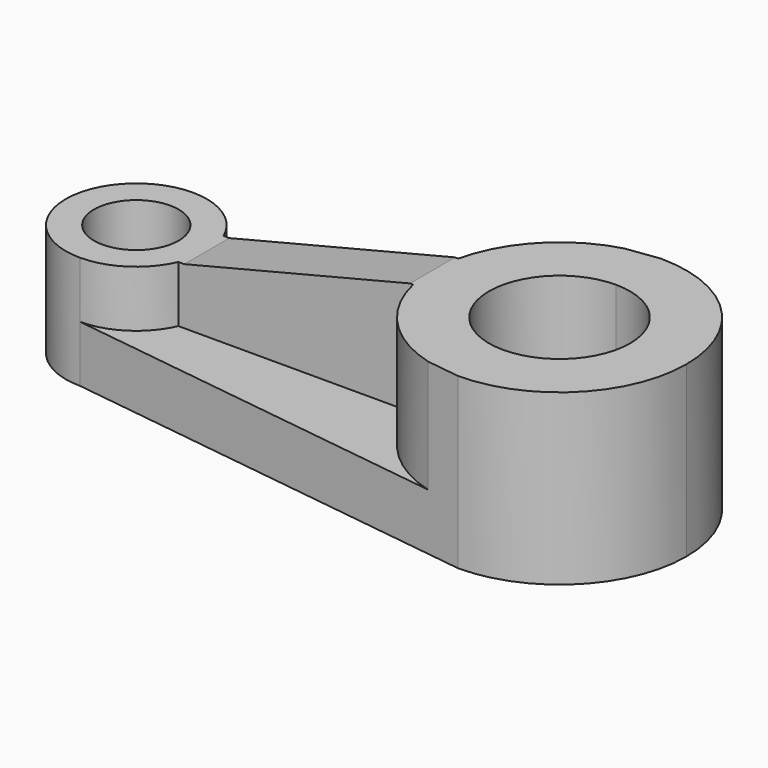
from build123d import *

# Parameters (mm, degrees)
F1_DEPTH = 25.4
F2_DEPTH = 38.1
F3_DEPTH = 12.7
F5_DEPTH = 6.35


with BuildPart() as f1:
    # F0 (on Top) → F1 (new body)
    with BuildSketch(Plane.XY):
        with BuildLine():
            ThreePointArc((-50.8001835883, 0), (-55.449863437, 11.2253201513), (-66.6751835883, 15.875))
            Line((-66.6751835883, 15.875), (-66.6751835883, 9.525))
            ThreePointArc((-66.6751835883, 9.525), (-59.9399914975, 6.7351920908), (-57.1501835883, 0))
            ThreePointArc((-57.1501835883, 0), (-59.9399914975, -6.7351920908), (-66.6751835883, -9.525))
            Line((-66.6751835883, -9.525), (-66.6751835883, -15.875))
            ThreePointArc((-66.6751835883, -15.875), (-55.449863437, -11.2253201513), (-50.8001835883, 0))
        make_face()
        with BuildLine():
            Line((-66.6751835883, 9.525), (-66.6751835883, 15.875))
            ThreePointArc((-66.6751835883, 15.875), (-82.5501835883, 0), (-66.6751835883, -15.875))
            Line((-66.6751835883, -15.875), (-66.6751835883, -9.525))
            ThreePointArc((-66.6751835883, -9.525), (-76.2001835883, 0), (-66.6751835883, 9.525))
        make_face()
    extrude(amount=F1_DEPTH)



with BuildPart() as f2:
    # F0 (on Top) → F2 (new body)
    with BuildSketch(Plane.XY):
        with BuildLine():
            ThreePointArc((28.5748164117, -15.875), (12.6998164117, 0), (28.5748164117, 15.875))
            Line((28.5748164117, 15.875), (28.5748164117, 28.575))
            Line((28.5748164117, 28.575), (21.0879168484, 27.5767467249))
            ThreePointArc((21.0879168484, 27.5767467249), (-0.0001835883, 0), (21.0879168484, -27.5767467249))
            Line((21.0879168484, -27.5767467249), (28.5748164117, -28.575))
            Line((28.5748164117, -28.575), (28.5748164117, -15.875))
        make_face()
        with BuildLine():
            ThreePointArc((28.5748164117, 15.875), (39.800136563, 11.2253201513), (44.4498164117, 0))
            ThreePointArc((44.4498164117, 0), (39.800136563, -11.2253201513), (28.5748164117, -15.875))
            Line((28.5748164117, -15.875), (28.5748164117, -28.575))
            ThreePointArc((28.5748164117, -28.575), (48.7803926841, -20.2055762724), (57.1498164117, 0))
            ThreePointArc((57.1498164117, 0), (48.7803926841, 20.2055762724), (28.5748164117, 28.575))
            Line((28.5748164117, 28.575), (28.5748164117, 15.875))
        make_face()
    extrude(amount=F2_DEPTH)


with BuildPart() as f1_1:
    add(f1.part)

    add(f2.part)  # F3 merges F2
    # F0 (on Top) → F3 (join)
    with BuildSketch(Plane.XY):
        with BuildLine():
            ThreePointArc((21.0879168484, -27.5767467249), (-0.0001835883, 0), (21.0879168484, 27.5767467249))
            Line((21.0879168484, 27.5767467249), (-66.6751835883, 15.875))
            ThreePointArc((-66.6751835883, 15.875), (-55.449863437, 11.2253201513), (-50.8001835883, 0))
            ThreePointArc((-50.8001835883, 0), (-55.449863437, -11.2253201513), (-66.6751835883, -15.875))
            Line((-66.6751835883, -15.875), (21.0879168484, -27.5767467249))
        make_face()
    extrude(amount=F3_DEPTH)

    # F4 (on Front) → F5 (join, symmetric)
    with BuildSketch(Plane.XZ):
        Polygon((-50.8, 0), (0, 0), (4.6227602288, 0), (4.6227602288, 38.1), (0, 38.1), (-50.8, 25.4), (-54.4934645295, 25.4), (-54.4934645295, 0), align=None)
    extrude(amount=F5_DEPTH, both=True)


solid = f1_1.part
